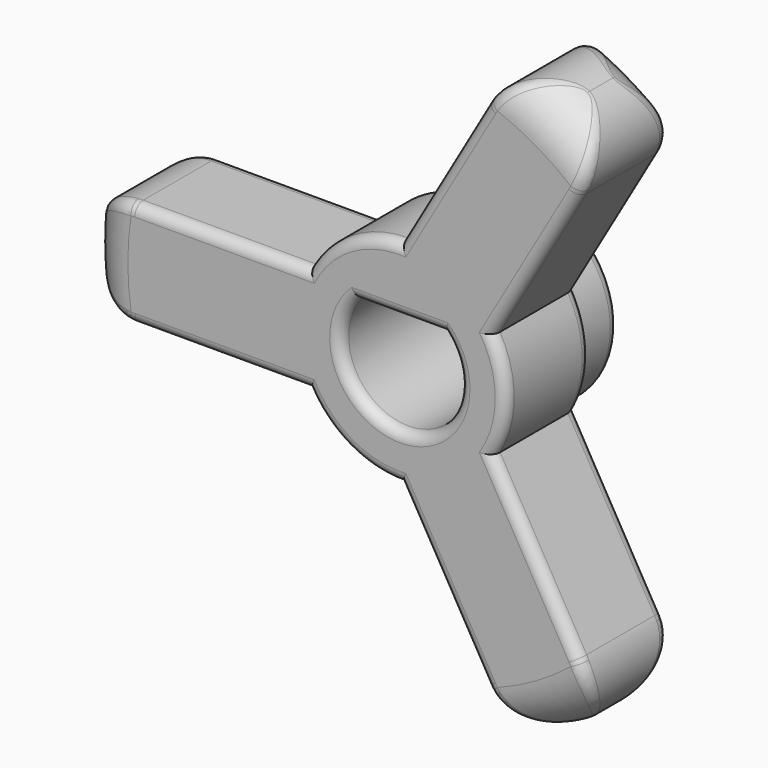
from build123d import *

# Parameters (mm, degrees)
F1_DEPTH = 19.05
F3_DEPTH = 19.051
F7_R     = 1.269


# Not quite as in the source:
# - a fillet or chamfer is up to 0.001 mm smaller than in the source, because OpenCascade refuses the exact size


with BuildPart() as f1:
    # F0 (on Front) → F1 (new body)
    with BuildSketch(Plane.XZ):
        with BuildLine():
            Line((-31.75, -6.35), (-10.9985226281, -6.35))
            ThreePointArc((-10.9985226281, -6.35), (-6.35, -10.9985226281), (0, -12.7))
            Line((0, -12.7), (10.375738686, -30.6713065702))
            ThreePointArc((10.375738686, -30.6713065702), (14.2314990636, -33.6299355671), (19.05, -32.9955678842))
            ThreePointArc((19.05, -32.9955678842), (22.0086289969, -29.1398075066), (21.374261314, -24.3213065702))
            Line((21.374261314, -24.3213065702), (10.9985226281, -6.35))
            ThreePointArc((10.9985226281, -6.35), (12.7, 0), (10.9985226281, 6.35))
            Line((10.9985226281, 6.35), (21.374261314, 24.3213065702))
            ThreePointArc((21.374261314, 24.3213065702), (22.0086289969, 29.1398075066), (19.05, 32.9955678842))
            ThreePointArc((19.05, 32.9955678842), (14.2314990636, 33.6299355671), (10.375738686, 30.6713065702))
            Line((10.375738686, 30.6713065702), (0, 12.7))
            ThreePointArc((0, 12.7), (-6.35, 10.9985226281), (-10.9985226281, 6.35))
            Line((-10.9985226281, 6.35), (-31.75, 6.35))
            ThreePointArc((-31.75, 6.35), (-36.2401280605, 4.4901280605), (-38.1, 0))
            ThreePointArc((-38.1, 0), (-36.2401280605, -4.4901280605), (-31.75, -6.35))
        make_face()
    extrude(amount=F1_DEPTH)

    # F2 (on face) → F3 (cut, through all)
    with BuildSketch(Plane.XZ.offset(19.05)):
        with BuildLine():
            Line((5.2351119186, 4.8514), (-5.2351119186, 4.8514))
            ThreePointArc((-5.2351119186, 4.8514), (0, -7.1374), (5.2351119186, 4.8514))
        make_face()
    extrude(amount=-F3_DEPTH, mode=Mode.SUBTRACT)

    # F4 (on Top) → F6 (revolve, cut)
    with BuildSketch(Plane.XY):
        with BuildLine():
            Line((-10.9985226281, -25.4), (-10.9985226281, -19.05))
            Line((-10.9985226281, -19.05), (-32.5885226281, -19.05))
            ThreePointArc((-32.5885226281, -19.05), (-36.3103152121, -17.6455897546), (-38.1765226281, -14.13256))
            Line((-38.1765226281, -14.13256), (-38.1765226281, -25.4))
            Line((-38.1765226281, -25.4), (-10.9985226281, -25.4))
        make_face()
        with BuildLine():
            Line((-32.5885226281, -6.35), (-10.9985226281, -6.35))
            Line((-10.9985226281, -6.35), (-10.9985226281, 0))
            Line((-10.9985226281, 0), (-38.1765226281, 0))
            Line((-38.1765226281, 0), (-38.1765226281, -11.26744))
            ThreePointArc((-38.1765226281, -11.26744), (-36.3103152121, -7.7544102454), (-32.5885226281, -6.35))
        make_face()
    revolve(axis=Axis((0, 0, 0), (0, 1, 0)), mode=Mode.SUBTRACT)

    # F7 (radius 1.27 in the source; OpenCascade refuses exactly that, so slightly less here)
    f7_edges = [f1.edges().sort_by_distance(p)[0] for p in [
        (10.998523, 0, 0),
        (0, 0, 4.8514),
        (0, 0, -7.1374),
        (0, -19.05, -7.1374),
        (-6.35, -19.05, -10.998523),
        (-21.374261, -19.05, -6.35),
        (5.187869, -19.05, -21.685653),
        (16.186392, -19.05, -15.335653),
        (12.7, -19.05, 0),
        (0, -19.05, 4.8514),
        (-6.35, -19.05, 10.998523),
        (-21.374261, -19.05, 6.35),
        (5.187869, -19.05, 21.685653),
        (16.186392, -19.05, 15.335653),
        (-21.374261, -6.35, -6.35),
        (-21.374261, -6.35, 6.35),
        (-6.35, -6.35, -10.998523),
        (5.187869, -6.35, -21.685653),
        (16.186392, -6.35, -15.335653),
        (16.186392, -6.35, 15.335653),
        (12.7, -6.35, 0),
        (5.187869, -6.35, 21.685653),
        (-6.35, -6.35, 10.998523),
        (21.427132, -6.35, 24.414696),
        (19.05458, -10.816485, 32.992921),
        (10.430181, -6.35, 30.763789),
        (10.430181, -19.05, 30.763789),
        (19.045418, -14.583515, 32.998211),
        (21.427132, -19.05, 24.414696),
        (10.430181, -6.35, -30.763789),
        (19.045418, -10.816485, -32.998211),
        (21.427132, -6.35, -24.414696),
        (21.427132, -19.05, -24.414696),
        (19.05458, -14.583515, -32.992921),
        (10.430181, -19.05, -30.763789),
        (-31.857313, -19.05, 6.349093),
        (-31.857313, -19.05, -6.349093),
        (-38.1, -14.583507, 0),
        (-31.857313, -6.35, 6.349093),
        (-31.857313, -6.35, -6.349093),
        (-38.099997, -10.816482, 0.005944),
    ]]
    fillet(f7_edges, radius=F7_R)


solid = f1.part
